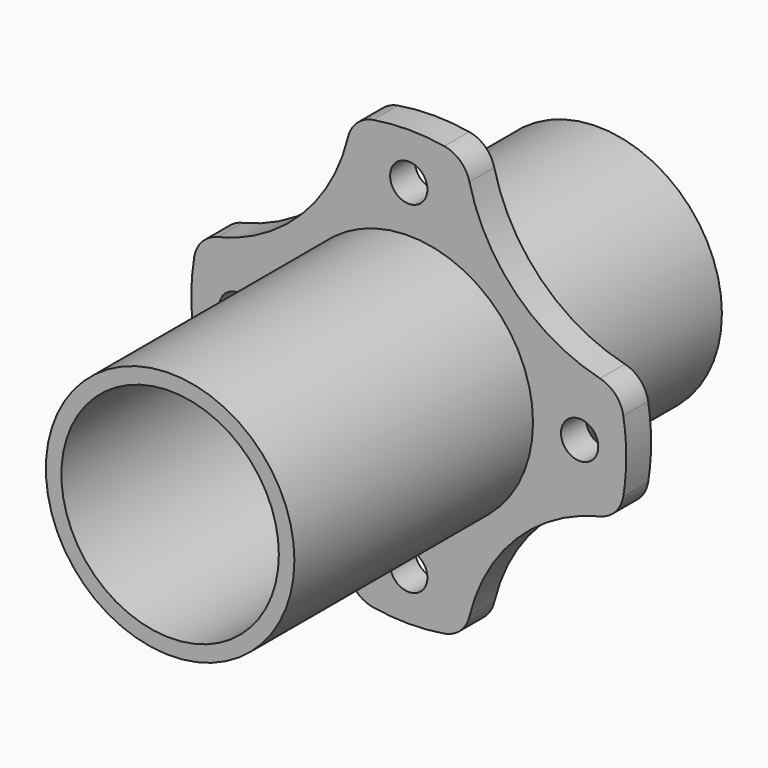
from build123d import *

# Parameters (mm, degrees)
F1_R     = 25.4
F1_R_2   = 22.225
F2_DEPTH = 54.61
F3_R     = 3.81
F3_R_2   = 25.4
F4_DEPTH = 3.175
F5_R     = 6.35


with BuildPart() as f2:
    # F1 (on offset) → F2 (new body, symmetric)
    with BuildSketch(Plane.XZ.offset(9.525)):
        Circle(F1_R)
        Circle(F1_R_2, mode=Mode.SUBTRACT)
    extrude(amount=F2_DEPTH, both=True)

    # F3 (on Front) → F4 (join, symmetric)
    with BuildSketch(Plane.XZ):
        with BuildLine():
            ThreePointArc((42.8826136347, -11.6997413585), (44.0564108619, -5.902131985), (44.45, 0))
            ThreePointArc((44.45, 0), (44.0564108619, 5.902131985), (42.8826136347, 11.6997413585))
            ThreePointArc((42.8826136347, 11.6997413585), (22.0016274966, 22.0016274966), (11.6997413585, 42.8826136347))
            ThreePointArc((11.6997413585, 42.8826136347), (0, 44.45), (-11.6997413585, 42.8826136347))
            ThreePointArc((-11.6997413585, 42.8826136347), (-22.0016274966, 22.0016274966), (-42.8826136347, 11.6997413585))
            ThreePointArc((-42.8826136347, 11.6997413585), (-44.45, 0), (-42.8826136347, -11.6997413585))
            ThreePointArc((-42.8826136347, -11.6997413585), (-22.0016274966, -22.0016274966), (-11.6997413585, -42.8826136347))
            ThreePointArc((-11.6997413585, -42.8826136347), (0, -44.45), (11.6997413585, -42.8826136347))
            ThreePointArc((11.6997413585, -42.8826136347), (22.0016274966, -22.0016274966), (42.8826136347, -11.6997413585))
        make_face()
        with Locations((0, -34.925)):
            Circle(F3_R, mode=Mode.SUBTRACT)
        with Locations((-34.925, 0)):
            Circle(F3_R, mode=Mode.SUBTRACT)
        Circle(F3_R_2, mode=Mode.SUBTRACT)
        with Locations((34.925, 0)):
            Circle(F3_R, mode=Mode.SUBTRACT)
        with Locations((0, 34.925)):
            Circle(F3_R, mode=Mode.SUBTRACT)
    extrude(amount=F4_DEPTH, both=True)

    # F5
    f5_edges = [f2.edges().sort_by_distance(p)[0] for p in [
        (11.699741, 0, 42.882614),
        (-42.882614, 0, 11.699741),
        (-11.699741, 0, -42.882614),
        (42.882614, 0, -11.699741),
        (42.882614, 0, 11.699741),
        (-11.699741, 0, 42.882614),
        (-42.882614, 0, -11.699741),
        (11.699741, 0, -42.882614),
    ]]
    fillet(f5_edges, radius=F5_R)


solid = f2.part
